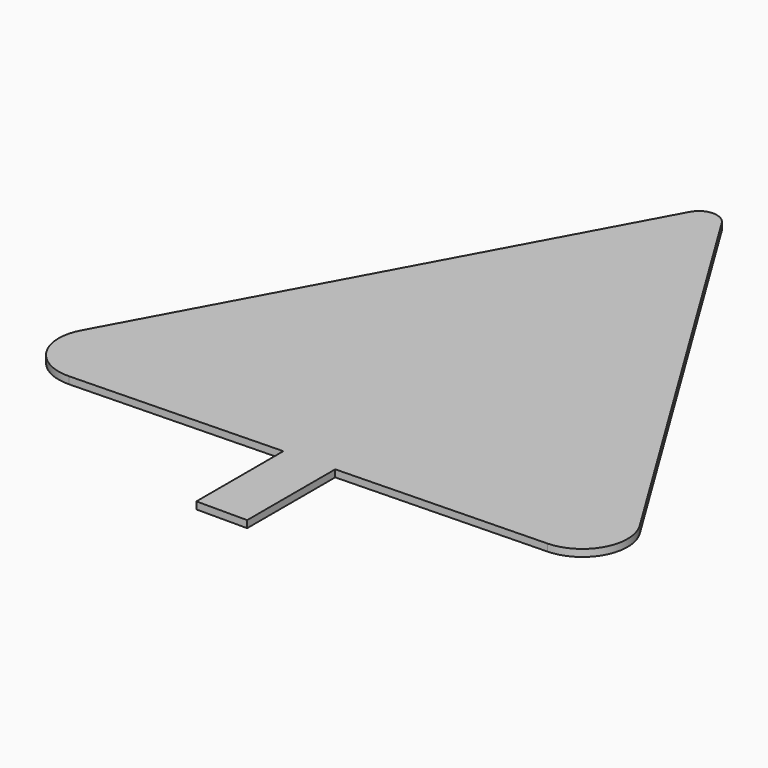
from build123d import *

# Parameters (mm, degrees)
F1_DEPTH = 1


# Not quite as in the source:
# - a feature names something its author has since deleted; it is built from what else it names


with BuildPart() as f1:
    # F0 (on Top) → F1 (new body)
    with BuildSketch(Plane.XY):
        with BuildLine():
            Line((-2.7494849637, -25.4823859731), (-2.7494849637, -25.250749146))
            ThreePointArc((-2.7494849637, -25.250749146), (-22.497868801, -11.7900763108), (-22.3279049811, 12.1088669642))
            Line((-22.3279049811, 12.1088669642), (-38.057784897, -16.8959317215))
            ThreePointArc((-38.057784897, -16.8959317215), (-37.8884434924, -23.2436733268), (-32.3064673032, -26.2708901713))
            Line((-32.3064673032, -26.2708901713), (-2.7494849637, -25.4823859731))
        make_face()
        with BuildLine():
            ThreePointArc((25.4, 0), (19.4537790742, -16.3312730591), (4.3991748244, -25.0161400073))
            Line((4.3991748244, -25.0161400073), (4.3991748244, -25.2916781332))
            Line((4.3991748244, -25.2916781332), (33.6611985399, -24.5110426718))
            ThreePointArc((33.6611985399, -24.5110426718), (39.0738333245, -21.1905179108), (38.9044919199, -14.8427763054))
            Line((38.9044919199, -14.8427763054), (21.6505391613, 13.2820990068))
            ThreePointArc((21.6505391613, 13.2820990068), (24.4446690988, 6.9005907466), (25.4, 0))
        make_face()
        with BuildLine():
            ThreePointArc((-22.3279049811, 12.1088669642), (-22.497868801, -11.7900763108), (-2.7494849637, -25.250749146))
            ThreePointArc((-2.7494849637, -25.250749146), (0.8331443579, -25.3863323558), (4.3991748244, -25.0161400073))
            ThreePointArc((4.3991748244, -25.0161400073), (19.4537790742, -16.3312730591), (25.4, 0))
            ThreePointArc((25.4, 0), (24.4446690988, 6.9005907466), (21.6505391613, 13.2820990068))
            ThreePointArc((21.6505391613, 13.2820990068), (-0.6773658317, 25.3909664158), (-22.3279049811, 12.1088669642))
        make_face()
        with BuildLine():
            Line((-3.4520485887, 46.9146262965), (-22.3279049811, 12.1088669642))
            ThreePointArc((-22.3279049811, 12.1088669642), (-0.6773658317, 25.3909664158), (21.6505391613, 13.2820990068))
            Line((21.6505391613, 13.2820990068), (0.9457958008, 47.0319494631))
            ThreePointArc((0.9457958008, 47.0319494631), (-1.2869946749, 48.2428362009), (-3.4520485887, 46.9146262965))
        make_face()
        with BuildLine():
            ThreePointArc((4.3991748244, -25.0161400073), (0.8331443579, -25.3863323558), (-2.7494849637, -25.250749146))
            Line((-2.7494849637, -25.250749146), (-2.7494849637, -25.4823859731))
            Line((-2.7494849637, -25.4823859731), (-2.7494849637, -40.7840199769))
            Line((-2.7494849637, -40.7840199769), (4.3991748244, -40.7840199769))
            Line((4.3991748244, -40.7840199769), (4.3991748244, -25.2916781332))
            Line((4.3991748244, -25.2916781332), (4.3991748244, -25.0161400073))
        make_face()
    extrude(amount=F1_DEPTH)


solid = f1.part
